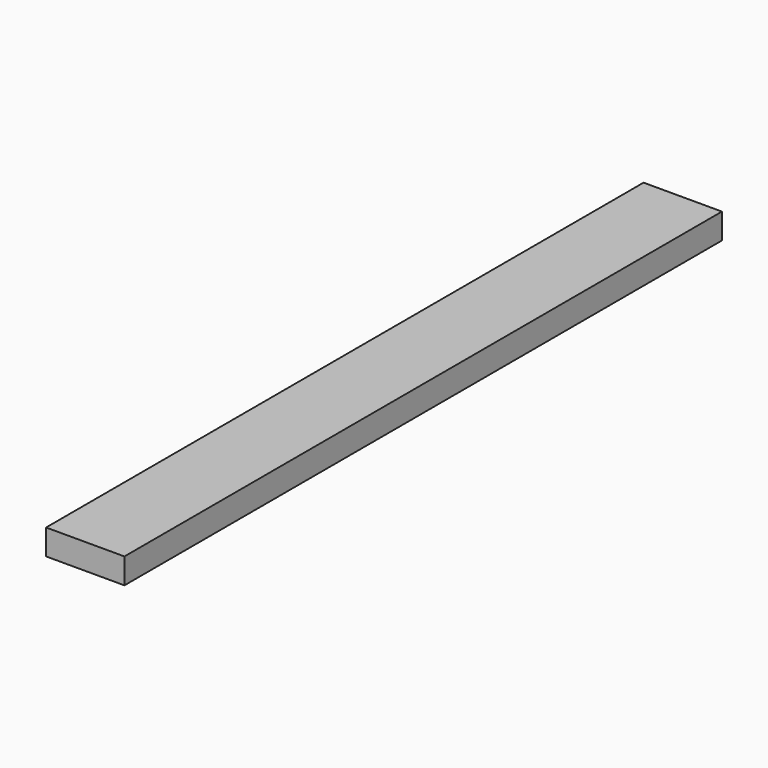
from build123d import *

# Parameters (mm, degrees)
F1_E0_W  = 12589.5175933838
F1_E0_H  = 120000
F2_DEPTH = 4094


with BuildPart() as f2:
    # F1_E0 (on explicit) → F2 (new body)
    with BuildSketch(Plane(origin=(0, 0, 0), x_dir=(1, 0, 0), z_dir=(0, 0, -1))):
        with Locations((6294.7587966919, 60000)):
            Rectangle(F1_E0_W, F1_E0_H)
    extrude(amount=-F2_DEPTH)


solid = f2.part
